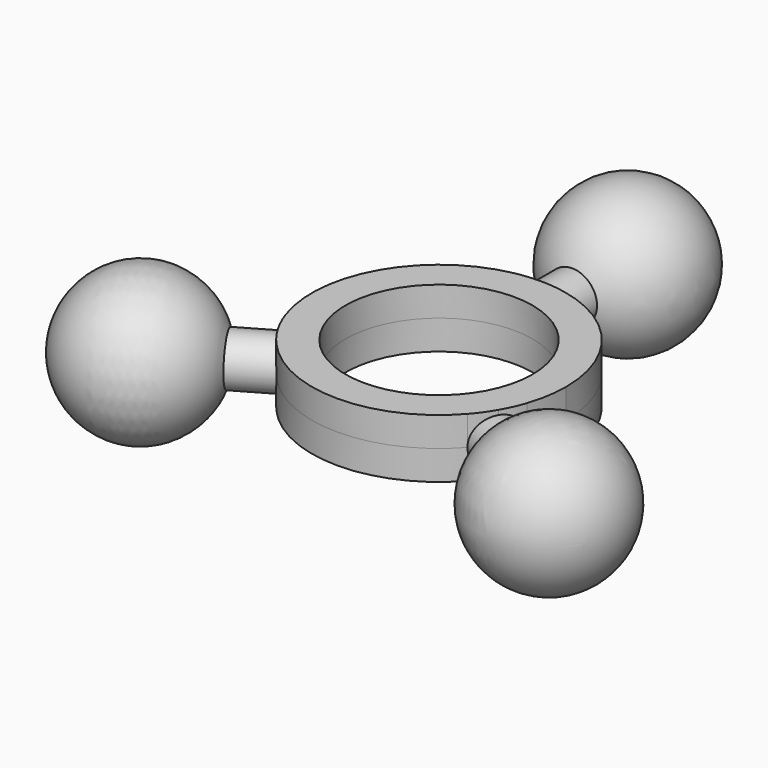
from build123d import *

# Parameters (mm, degrees)
F1_DEPTH = 3.5


# Not quite as in the source:
# - a feature names something its author has since deleted; it is built from what else it names


with BuildPart() as f1:
    # F0 (on Top) → F1 (new body, symmetric)
    with BuildSketch(Plane.XY):
        with BuildLine():
            ThreePointArc((11.1, 0), (-6.7057978456, -8.8454663672), (-2.9977072529, 10.6875512268))
            Line((-2.9977072529, 10.6875512268), (-2.9977072529, 14.7994510447))
            ThreePointArc((-2.9977072529, 14.7994510447), (-13.0888974447, 7.5293269077), (-14.300301744, -4.8488524447))
            ThreePointArc((-14.300301744, -4.8488524447), (-13.7551076947, -6.2295274547), (-13.0769835971, -7.55))
            ThreePointArc((-13.0769835971, -7.55), (-12.2574966376, -8.8183771851), (-11.3154218332, -9.9985613333))
            ThreePointArc((-11.3154218332, -9.9985613333), (0.0220311162, -15.0999839281), (11.3445497157, -9.9655000751))
            ThreePointArc((11.3445497157, -9.9655000751), (12.2703497298, -8.8004839361), (13.0769835971, -7.55))
            ThreePointArc((13.0769835971, -7.55), (13.7641811407, -6.2094538831), (14.3143885689, -4.8071072278))
            ThreePointArc((14.3143885689, -4.8071072278), (14.9023029662, -2.4354396533), (15.1, 0))
            ThreePointArc((15.1, 0), (11.6752542258, 9.5759301774), (2.9545114222, 14.8081350026))
            Line((2.9545114222, 14.8081350026), (2.9545114222, 10.6995729941))
            ThreePointArc((2.9545114222, 10.6995729941), (8.8319045734, 6.7236494262), (11.1, 0))
        make_face()
        with BuildLine():
            Line((-2.9977072529, 14.7994510447), (-2.9977072529, 10.6875512268))
            ThreePointArc((-2.9977072529, 10.6875512268), (-0.0224187571, 11.0999773603), (2.9545114222, 10.6995729941))
            Line((2.9545114222, 10.6995729941), (2.9545114222, 14.8081350026))
            ThreePointArc((2.9545114222, 14.8081350026), (1.4844462705, 15.0268565998), (0, 15.1))
            ThreePointArc((0, 15.1), (-1.5063680202, 15.0246748846), (-2.9977072529, 14.7994510447))
        make_face()
    extrude(amount=F1_DEPTH, both=True)



with BuildPart() as f2:
    # F0 (on Top) → F2 (revolve)
    with BuildSketch(Plane.XY):
        with BuildLine():
            ThreePointArc((-16.6773661399, -9.6286818303), (-17.5385305233, -8.3965794521), (-18.5978756937, -7.3300579213))
            ThreePointArc((-18.5978756937, -7.3300579213), (-29.8607484047, -7.2897269682), (-31.8328094306, -18.3786810938))
            Line((-31.8328094306, -18.3786810938), (-29.667745666, -17.1286809465))
            ThreePointArc((-29.667745666, -17.1286809465), (-27.378292812, -8.5941316732), (-18.8424299045, -10.8786819775))
            Line((-18.8424299045, -10.8786819775), (-16.6773661399, -9.6286818303))
        make_face()
    revolve(axis=Axis((-21.9539075231, -12.6750944182, 0), (-0.8660254038, -0.5, 0)))


with BuildPart() as f3:
    # F0 (on Top) → F3 (revolve)
    with BuildSketch(Plane.XY):
        with BuildLine():
            Line((18.8424299045, -10.8786819775), (16.6773661399, -9.6286818303))
            ThreePointArc((16.6773661399, -9.6286818303), (16.0385620789, -10.9933706318), (15.6433642715, -12.4474218161))
            ThreePointArc((15.6433642715, -12.4474218161), (21.243243587, -22.2227568333), (31.8328094306, -18.3786810938))
            Line((31.8328094306, -18.3786810938), (29.667745666, -17.1286809465))
            ThreePointArc((29.667745666, -17.1286809465), (21.128292812, -19.4194492205), (18.8424299045, -10.8786819775))
        make_face()
    revolve(axis=Axis((21.9539075231, -12.6750944182, 0), (0.8660254038, -0.5, 0)))


with BuildPart() as f4:
    # F0 (on Top) → F4 (revolve)
    with BuildSketch(Plane.XY):
        with BuildLine():
            ThreePointArc((0, 19.2511449544), (1.4994357076, 19.3805769593), (2.9545114222, 19.7650437981))
            ThreePointArc((2.9545114222, 19.7650437981), (8.6205679951, 29.5005806621), (0, 36.7511449544))
            Line((0, 36.7511449544), (0, 34.2511449544))
            ThreePointArc((0, 34.2511449544), (6.25, 28.0011449544), (0, 21.7511449544))
            Line((0, 21.7511449544), (0, 19.2511449544))
        make_face()
    revolve(axis=Axis((0, 25.3501888365, 0), (0, 1, 0)))


with BuildPart() as f1_1:
    add(f1.part)

    add(f4.part)  # F5 merges F4
    # F0 (on Top) → F5 (revolve)
    with BuildSketch(Plane.XY):
        with BuildLine():
            ThreePointArc((0, 15.1), (1.4844462705, 15.0268565998), (2.9545114222, 14.8081350026))
            Line((2.9545114222, 14.8081350026), (2.9545114222, 19.7650437981))
            ThreePointArc((2.9545114222, 19.7650437981), (1.4994357076, 19.3805769593), (0, 19.2511449544))
            Line((0, 19.2511449544), (0, 15.1))
        make_face()
    revolve(axis=Axis((0, 25.3501888365, 0), (0, 1, 0)))


    add(f3.part)  # F6 merges F3
    # F0 (on Top) → F6 (revolve)
    with BuildSketch(Plane.XY):
        with BuildLine():
            Line((16.6773661399, -9.6286818303), (13.0769835971, -7.55))
            ThreePointArc((13.0769835971, -7.55), (12.2703497298, -8.8004839361), (11.3445497157, -9.9655000751))
            Line((11.3445497157, -9.9655000751), (15.6433642715, -12.4474218161))
            ThreePointArc((15.6433642715, -12.4474218161), (16.0385620789, -10.9933706318), (16.6773661399, -9.6286818303))
        make_face()
    revolve(axis=Axis((21.9539075231, -12.6750944182, 0), (0.8660254038, -0.5, 0)))


    add(f2.part)  # F7 merges F2
    # F0 (on Top) → F7 (revolve)
    with BuildSketch(Plane.XY):
        with BuildLine():
            ThreePointArc((-13.0769835971, -7.55), (-13.7551076947, -6.2295274547), (-14.300301744, -4.8488524447))
            Line((-14.300301744, -4.8488524447), (-18.5978756937, -7.3300579213))
            ThreePointArc((-18.5978756937, -7.3300579213), (-17.5385305233, -8.3965794521), (-16.6773661399, -9.6286818303))
            Line((-16.6773661399, -9.6286818303), (-13.0769835971, -7.55))
        make_face()
    revolve(axis=Axis((-21.9539075231, -12.6750944182, 0), (-0.8660254038, -0.5, 0)))


solid = f1_1.part
